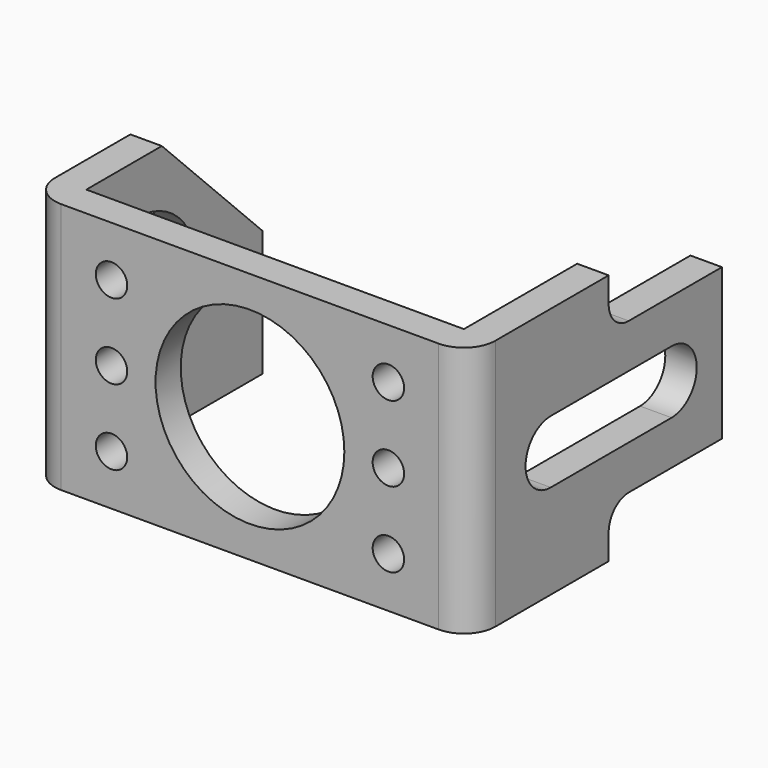
from build123d import *

# Parameters (mm, degrees)
F0_W        = 35
F0_H        = 20
F1_DEPTH    = 20
F2_W        = 30
F2_H        = 17.5
F3_DEPTH    = 25
F4_R        = 6
F5_DEPTH    = 5
F6_T1_DEPTH = 32.5
F7_R        = 7.5
F7_R_2      = 1.25
F8_DEPTH    = 25
F9_R        = 1.25
F10_DEPTH   = 25
F11_DEPTH   = 5
F13_DEPTH   = 5


# Not quite as in the source:
# - a fillet or chamfer that OpenCascade refuses, or shapes differently, is made with other operations: its cross-section is extruded or revolved along the edge and cut away or added


with BuildPart() as f1:
    # F0 (on Top) → F1 (new body)
    with BuildSketch(Plane.XY):
        with Locations((17.5, 10)):
            Rectangle(F0_W, F0_H)
    extrude(amount=F1_DEPTH)

    # F2 (on face) → F3 (cut)
    with BuildSketch(Plane.XY.offset(20)):
        with Locations((17.5, 11.25)):
            Rectangle(F2_W, F2_H)
    extrude(amount=-F3_DEPTH, mode=Mode.SUBTRACT)

    # F4 (on face) → F5 (cut)
    with BuildSketch(Plane(origin=(0, 0, 0), x_dir=(0, -1, 0), z_dir=(-1, 0, 0))):
        with Locations((-7.5, 10)):
            Circle(F4_R)
        Polygon((-20, 20), (-20, 10), (-10, 20), align=None)
    extrude(amount=-F5_DEPTH, mode=Mode.SUBTRACT)

    # F6: fillet of radius 2.5 on 2 edges, made by hand

    # F6_s2 → F6_t1 (cut)
    with BuildSketch(Plane.XY.offset(-6.25)):
        with BuildLine():
            ThreePointArc((0, 2.5), (0.732233047, 0.732233047), (2.5, 0))
            Line((2.5, 0), (0, 0))
            Line((0, 0), (0, 2.5))
        make_face()
        with BuildLine():
            ThreePointArc((32.5, 0), (34.267766953, 0.732233047), (35, 2.5))
            Line((35, 2.5), (35, 0))
            Line((35, 0), (32.5, 0))
        make_face()
    extrude(amount=F6_T1_DEPTH, mode=Mode.SUBTRACT)

    # F7 (on face) → F8 (cut)
    with BuildSketch(Plane.XZ):
        with Locations((17.5, 10)):
            Circle(F7_R)
        with Locations((28.5, 16)):
            Circle(F7_R_2)
        with Locations((28.5, 10)):
            Circle(F7_R_2)
        with Locations((28.5, 4)):
            Circle(F7_R_2)
    extrude(amount=-F8_DEPTH, mode=Mode.SUBTRACT)

    # F9 (on face) → F10 (cut)
    with BuildSketch(Plane.XZ):
        with Locations((6.5, 4)):
            Circle(F9_R)
        with Locations((6.5, 10)):
            Circle(F9_R)
        with Locations((6.5, 16)):
            Circle(F9_R)
    extrude(amount=-F10_DEPTH, mode=Mode.SUBTRACT)

    # F11 (add): a face of the model
    f11_faces = [f1.faces().sort_by_distance(p)[0] for p in [
        (33.75, 20, 10),
    ]]
    extrude(f11_faces, amount=F11_DEPTH)

    # F12 (on face) → F13 (cut)
    with BuildSketch(Plane.YZ.offset(35)):
        with BuildLine():
            Line((8, 7.5), (20, 7.5))
            ThreePointArc((20, 7.5), (22.5, 10), (20, 12.5))
            Line((20, 12.5), (8, 12.5))
            ThreePointArc((8, 12.5), (5.5, 10), (8, 7.5))
        make_face()
        with BuildLine():
            Line((15.75, 16), (25, 16))
            Line((25, 16), (25, 20))
            Line((25, 20), (13.75, 20))
            Line((13.75, 20), (13.75, 18))
            ThreePointArc((13.75, 18), (14.3357864376, 16.5857864376), (15.75, 16))
        make_face()
        with BuildLine():
            Line((25, 0), (25, 4))
            Line((25, 4), (15.75, 4))
            ThreePointArc((15.75, 4), (14.3357864376, 3.4142135624), (13.75, 2))
            Line((13.75, 2), (13.75, 0))
            Line((13.75, 0), (25, 0))
        make_face()
    extrude(amount=-F13_DEPTH, mode=Mode.SUBTRACT)


solid = f1.part
